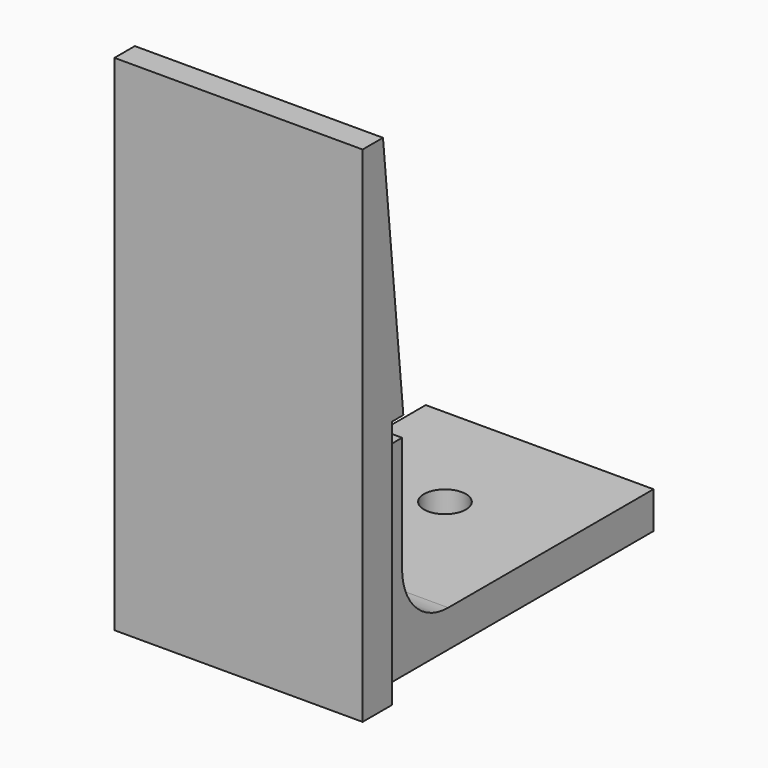
from build123d import *

# Parameters (mm, degrees)
F1_DEPTH      = 17.9
F0_W          = 2.9
F0_H          = 16.5
F0_H_2        = 1.5
F2_DEPTH      = 18
F2_DEPTH_BACK = 1.5
F4_D          = 3.3


# Not quite as in the source:
# - a feature names something its author has since deleted; it is built from what else it names


with BuildPart() as f1:
    # F0 (on Right) → F1 (new body)
    with BuildSketch(Plane.YZ):
        Polygon((3.4158524887, 16.5), (2.3158524887, 16.5), (2.3158524887, 0), (3.4158524887, 0), (3.4158524887, 7.4381744285), align=None)
        with BuildLine():
            ThreePointArc((7.9540269172, 2.9), (4.7450530046, 4.2292005159), (3.4158524887, 7.4381744285))
            Line((3.4158524887, 7.4381744285), (3.4158524887, 0))
            Line((3.4158524887, 0), (9.4158524887, 0))
            Line((9.4158524887, 0), (12.5158524887, 0))
            Line((12.5158524887, 0), (22.0158524887, 0))
            Line((22.0158524887, 0), (25.1158524887, 0))
            Line((25.1158524887, 0), (28.1158524887, 0))
            Line((28.1158524887, 0), (28.1158524887, 2.9))
            Line((28.1158524887, 2.9), (25.1158524887, 2.9))
            Line((25.1158524887, 2.9), (22.0158524887, 2.9))
            Line((22.0158524887, 2.9), (12.5158524887, 2.9))
            Line((12.5158524887, 2.9), (9.4158524887, 2.9))
            Line((9.4158524887, 2.9), (7.9540269172, 2.9))
        make_face()
    extrude(amount=F1_DEPTH)

    # F0 (on Right) → F2 (join, two sides)
    with BuildSketch(Plane.YZ) as f2_sk:
        with Locations((0.8658524887, 8.25)):
            Rectangle(F0_W, F0_H)
        Polygon((-0.5841475113, 18.1), (-0.5841475113, 16.5), (2.3158524887, 16.5), (2.3158524887, 18.1), (3.4158524887, 18.1), (1.4158524887, 38.1), (-0.5841475113, 38.1), align=None)
        with Locations((0.8658524887, -0.75)):
            Rectangle(F0_W, F0_H_2)
    extrude(amount=F2_DEPTH)
    extrude(f2_sk.sketch, amount=-F2_DEPTH_BACK)

    # F4 (through all)
    with Locations(Plane(origin=(0, 0, 0), x_dir=(1, 0, 0), z_dir=(0, 0, -1))):
        with Locations((8.95, -9.3158524887), (8.95, -18.8158524887)):
            Hole(F4_D / 2)


solid = f1.part
